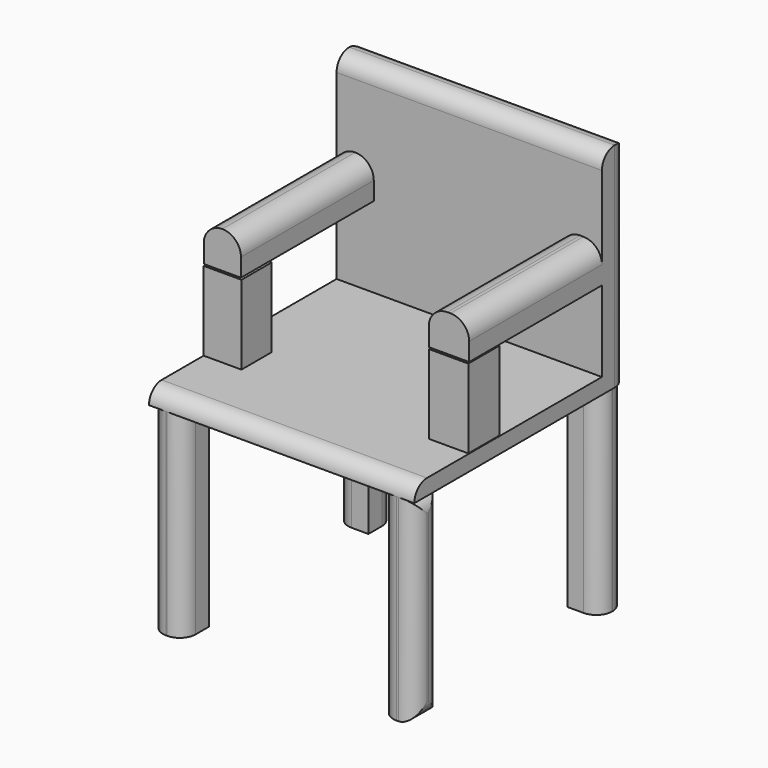
from build123d import *

# Parameters (mm, degrees)
F0_W      = 10.5122625828
F0_H      = 10.5122663081
F0_W_2    = 10.2786570787
F0_H_2    = 10.278660804
F0_H_3    = 10.5122625828
F0_W_3    = 10.7458680868
F0_H_4    = 10.7458718121
F1_DEPTH  = 63.5
F2_W      = 85.2661281824
F2_H      = 85.4979269207
F3_DEPTH  = 5.08
F4_W      = 85.2661281824
F4_H      = 10.16
F5_DEPTH  = 63.5
F7_W      = 12.1475029737
F7_H      = 12.1475029737
F7_W_2    = 12.6147139817
F7_H_2    = 12.6147139817
F8_DEPTH  = 25.4
F9_W      = 11.9528304785
F9_H      = 11.8126645684
F9_W_2    = 12.9729062319
F10_DEPTH = 53.34
F11_R     = 5.07999
F11_2_R   = 5.07999
F12_R     = 5.08
F13_R     = 5.969


# Not quite as in the source:
# - a fillet or chamfer is up to 0.001 mm smaller than in the source, because OpenCascade refuses the exact size


with BuildPart() as f1:
    # F0 (on Top) → F1 (new body)
    with BuildSketch(Plane.XY):
        with Locations((-37.0265245438, 37.1433291584)):
            Rectangle(F0_W, F0_H)
        with Locations((37.1433272958, 37.2601319104)):
            Rectangle(F0_W_2, F0_H_2)
        with Locations((-36.7929190397, -37.6105420291)):
            Rectangle(F0_W, F0_H_3)
        with Locations((37.3769327998, -37.4937374145)):
            Rectangle(F0_W_3, F0_H_4)
    extrude(amount=F1_DEPTH)

    # F11#2 (radius 5.08 in the source; OpenCascade refuses exactly that, so slightly less here)
    f11_2_edges = [f1.edges().sort_by_distance(p)[0] for p in [
        (-42.282656, 42.399462, 31.75),
        (-42.282656, 31.887196, 31.75),
        (-42.04905, -42.866673, 31.75),
        (-42.04905, -32.354411, 31.75),
        (-31.536788, -42.866673, 31.75),
        (32.003999, -42.866673, 31.75),
        (42.749867, -42.866673, 31.75),
        (42.749867, -32.120802, 31.75),
        (42.749867, -37.493737, 0),
        (42.749867, -37.493737, 63.5),
        (42.282656, 42.399462, 31.75),
        (42.282656, 32.120802, 31.75),
        (32.003999, 42.399462, 31.75),
    ]]
    fillet(f11_2_edges, radius=F11_2_R)

    # F12
    f12_edges = [f1.edges().sort_by_distance(p)[0] for p in [
        (32.003999, 37.319472, 31.75),
        (-31.770393, 42.399462, 31.75),
        (-37.202666, 42.399462, 31.75),
        (-42.282656, 37.319472, 31.75),
    ]]
    fillet(f12_edges, radius=F12_R)


with BuildPart() as f3:
    # F2 (on face) → F3 (new body)
    with BuildSketch(Plane.XY.offset(63.5)):
        with Locations((0.3504082561, -0.3495011479)):
            Rectangle(F2_W, F2_H)
    extrude(amount=F3_DEPTH)

    # F4 (on face) → F5 (join)
    with BuildSketch(Plane.XY.offset(68.58)):
        with Locations((0.3504082561, 37.3194623125)):
            Rectangle(F4_W, F4_H)
    extrude(amount=F5_DEPTH)

    # F7 (on face) → F8 (join)
    with BuildSketch(Plane.XY.offset(68.58)):
        with Locations((-36.2089043483, -15.065764077)):
            Rectangle(F7_W, F7_H)
        with Locations((36.4425098523, -14.832158573)):
            Rectangle(F7_W_2, F7_H_2)
    extrude(amount=F8_DEPTH)

    # F9 (on face) → F10 (join)
    with BuildSketch(Plane.XZ.offset(-32.2394623125)):
        with Locations((-36.3062405959, 100.4123203456)):
            Rectangle(F9_W, F9_H)
        with Locations((36.4970192313, 100.4123203456)):
            Rectangle(F9_W_2, F9_H)
    extrude(amount=F10_DEPTH)

    # F11 (radius 5.08 in the source; OpenCascade refuses exactly that, so slightly less here)
    f11_edges = [f3.edges().sort_by_distance(p)[0] for p in [
        (0.350408, -43.098465, 68.58),
        (0.350408, 32.239462, 132.08),
        (0.350408, 42.399462, 132.08),
        (42.983472, 42.399462, 97.79),
        (-42.282656, 42.399462, 97.79),
    ]]
    fillet(f11_edges, radius=F11_R)

    # F13
    f13_edges = [f3.edges().sort_by_distance(p)[0] for p in [
        (-42.282656, 5.569462, 106.318653),
        (-30.329825, 5.569462, 106.318653),
        (30.010566, 5.569462, 106.318653),
        (42.983472, 5.569462, 106.318653),
    ]]
    fillet(f13_edges, radius=F13_R)


solid = Compound([f1.part, f3.part])
